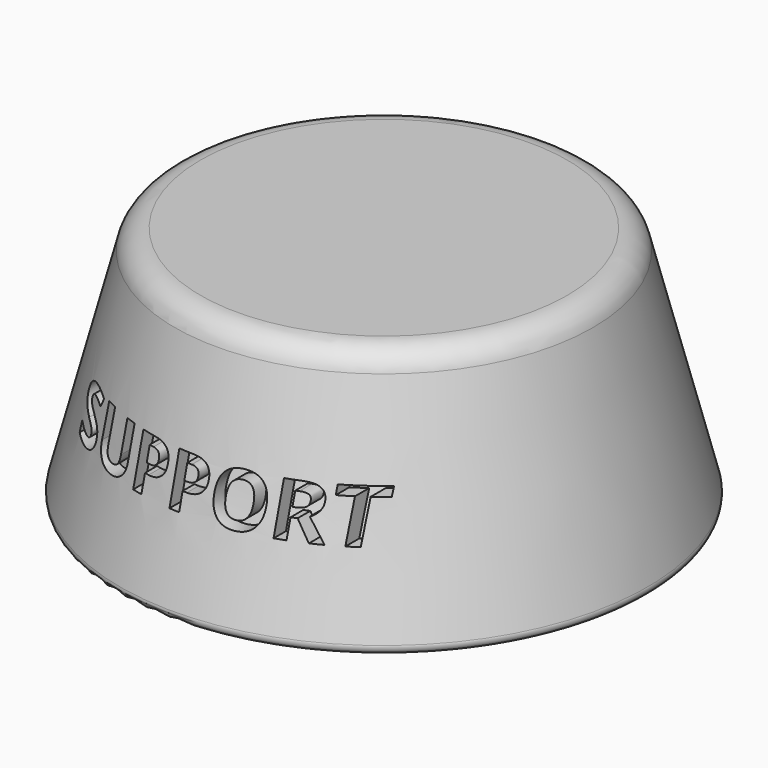
from build123d import *

# Parameters (mm, degrees)
F4_TEXT_SIZE = 7.538787736
F5_DEPTH     = 30.001
F9_R         = 3
F10_R        = 0.8


# Not quite as in the source:
# - Text() gives the source's letters only with a copy of the font that has no kerning and outlines rounded to 1/6400 em; it was checked with that copy


with BuildPart() as f1:
    # F0 (on Front) → F1 (revolve)
    with BuildSketch(Plane.XZ):
        Polygon((0, -19.987144978), (0, 7.012855022), (-23, 7.012855022), (-30, -19.987144978), align=None)
    revolve(axis=Axis((0, 0, -6.487144978), (0, 0, 1)))

    # F4 (on Front) → F5 (cut, through all)
    with BuildSketch(Plane.XZ):
        with Locations((-17.5, -10.4150721479)):
            Text('SUPPORT', F4_TEXT_SIZE, font='Open Sans', font_style=FontStyle.BOLD, text_align=(TextAlign.LEFT, TextAlign.BOTTOM))
    extrude(amount=F5_DEPTH, mode=Mode.SUBTRACT)

    # F6 (on Front) → F7 (revolve)
    with BuildSketch(Plane.XZ):
        Polygon((0, -19.987144978), (0, 7.012855022), (-21.3471021415, 7.012855022), (-28.3471021415, -19.987144978), align=None)
    revolve(axis=Axis((0, 0, -6.487144978), (0, 0, 1)))

    # F9
    f9_edges = [f1.edges().sort_by_distance(p)[0] for p in [
        (23, 0, 7.012855),
    ]]
    fillet(f9_edges, radius=F9_R)

    # F10
    f10_edges = [f1.edges().sort_by_distance(p)[0] for p in [
        (30, 0, -19.987145),
    ]]
    fillet(f10_edges, radius=F10_R)


solid = f1.part
